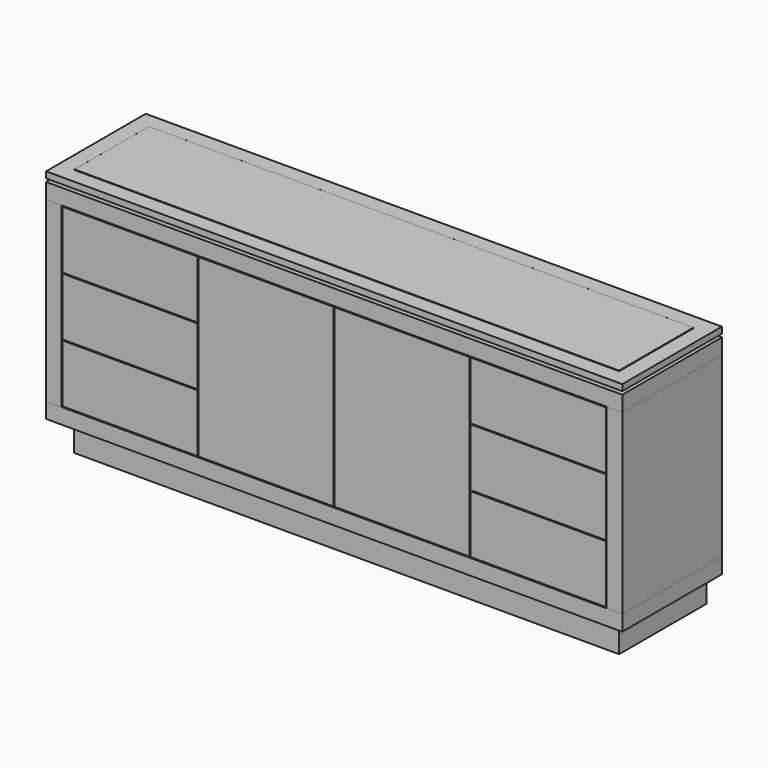
from build123d import *

# Parameters (mm, degrees)
F1_DEPTH  = 400
F0_W      = 50
F0_H      = 50
F0_W_2    = 1750
F0_H_2    = 570
F2_DEPTH  = 400
F3_START  = -50
F0_H_3    = 100
F3_DEPTH  = 350
F0_W_3    = 433.75
F0_H_4    = 186
F4_DEPTH  = 18
F0_H_5    = 3
F5_START  = -20
F5_DEPTH  = 360
F6_DEPTH  = 400
F9_W      = 1750
F9_H      = 300
F10_DEPTH = 5
F11_DEPTH = 6.5
F12_R     = 1.5


# Not quite as in the source:
# - a feature names something its author has since deleted; it is built from what else it names


with BuildPart() as f1:
    # F0 (on Front) → F1 (new body)
    with BuildSketch(Plane.XZ):
        Polygon((905, 770), (-875, 770), (-875, 720), (-872, 720), (875, 720), (925, 720), (925, 770), align=None)
        Polygon((-905, 770), (-925, 770), (-925, 720), (-875, 720), (-875, 770), align=None)
    extrude(amount=-F1_DEPTH)


with BuildPart() as f1b:
    # F0 (on Front) → F1, piece 2 (new body)
    with BuildSketch(Plane.XZ):
        with Locations((-900, 125)):
            Rectangle(F0_W, F0_H)
        with Locations((0, 125)):
            Rectangle(F0_W_2, F0_H)
        with Locations((900, 125)):
            Rectangle(F0_W, F0_H)
    extrude(amount=-F1_DEPTH)


with BuildPart() as f2:
    # F0 (on Front) → F2 (new body)
    with BuildSketch(Plane.XZ):
        with Locations((-900, 435)):
            Rectangle(F0_W, F0_H_2)
    extrude(amount=-F2_DEPTH)


with BuildPart() as f2b:
    # F0 (on Front) → F2, piece 2 (new body)
    with BuildSketch(Plane.XZ):
        with Locations((900, 435)):
            Rectangle(F0_W, F0_H_2)
    extrude(amount=-F2_DEPTH)


with BuildPart() as f3:
    # F0 (on Front) → F3 (new body)
    with BuildSketch(Plane.XZ.offset(F3_START)):
        with Locations((0, 50)):
            Rectangle(F0_W_2, F0_H_3)
    extrude(amount=-F3_DEPTH)


with BuildPart() as f4:
    # F0 (on Front) → F4 (new body)
    with BuildSketch(Plane.XZ):
        with Locations((-655.125, 435)):
            Rectangle(F0_W_3, F0_H_4)
    extrude(amount=-F4_DEPTH)


with BuildPart() as f4b:
    # F0 (on Front) → F4, piece 2 (new body)
    with BuildSketch(Plane.XZ):
        with Locations((-655.125, 246)):
            Rectangle(F0_W_3, F0_H_4)
    extrude(amount=-F4_DEPTH)


with BuildPart() as f4c:
    # F0 (on Front) → F4, piece 3 (new body)
    with BuildSketch(Plane.XZ):
        with Locations((-218.375, 435)):
            Rectangle(F0_W_3, F0_H_4)
        with Locations((-218.375, 246)):
            Rectangle(F0_W_3, F0_H_4)
        with Locations((-218.375, 340.5)):
            Rectangle(F0_W_3, F0_H_5)
        with Locations((-218.375, 624)):
            Rectangle(F0_W_3, F0_H_4)
        with Locations((-218.375, 529.5)):
            Rectangle(F0_W_3, F0_H_5)
    extrude(amount=-F4_DEPTH)


with BuildPart() as f4d:
    # F0 (on Front) → F4, piece 4 (new body)
    with BuildSketch(Plane.XZ):
        with Locations((-655.125, 624)):
            Rectangle(F0_W_3, F0_H_4)
    extrude(amount=-F4_DEPTH)


with BuildPart() as f5:
    # F0 (on Front) → F5 (new body)
    with BuildSketch(Plane.XZ.offset(F5_START)):
        Polygon((-905, 780), (-905, 770), (-875, 770), (905, 770), (905, 780), align=None)
    extrude(amount=-F5_DEPTH)


with BuildPart() as f6:
    # F0 (on Front) → F6 (new body)
    with BuildSketch(Plane.XZ):
        Polygon((-925, 780), (-905, 780), (905, 780), (925, 780), (925, 800), (-925, 800), align=None)
    extrude(amount=-F6_DEPTH)

    # F9 (on face) → F10 (cut)
    with BuildSketch(Plane.XY.offset(800)):
        with Locations((0, 200)):
            Rectangle(F9_W, F9_H)
    extrude(amount=-F10_DEPTH, mode=Mode.SUBTRACT)


with BuildPart() as f8_1:
    # F8: instance of F4d
    add(f4d.part.mirror(Plane(origin=(0, 9, 435), x_dir=(0, 1, 0), z_dir=(1, 0, 0))))


with BuildPart() as f8_2:
    # F8: instance of F4
    add(f4.part.mirror(Plane(origin=(0, 9, 435), x_dir=(0, 1, 0), z_dir=(1, 0, 0))))


with BuildPart() as f8_3:
    # F8: instance of F4b
    add(f4b.part.mirror(Plane(origin=(0, 9, 435), x_dir=(0, 1, 0), z_dir=(1, 0, 0))))


with BuildPart() as f8_4:
    # F8: instance of F4c
    add(f4c.part.mirror(Plane(origin=(0, 9, 435), x_dir=(0, 1, 0), z_dir=(1, 0, 0))))


with BuildPart() as f11:
    # F11 (new): a face of the model
    f11_faces = [f6.part.faces().sort_by_distance(p)[0] for p in [
        (0, 200, 795),
    ]]
    extrude(f11_faces, amount=F11_DEPTH)

    # F12
    f12_edges = [f11.edges().sort_by_distance(p)[0] for p in [
        (0, 350, 801.5),
        (-875, 200, 801.5),
        (0, 50, 801.5),
        (875, 200, 801.5),
        (-875, 50, 798.25),
        (-875, 350, 798.25),
        (875, 350, 798.25),
        (875, 50, 798.25),
    ]]
    fillet(f12_edges, radius=F12_R)


solid = Compound([f1.part, f1b.part, f2.part, f2b.part, f3.part, f4.part, f4b.part, f4c.part, f4d.part, f5.part, f6.part, f8_1.part, f8_2.part, f8_3.part, f8_4.part, f11.part])
